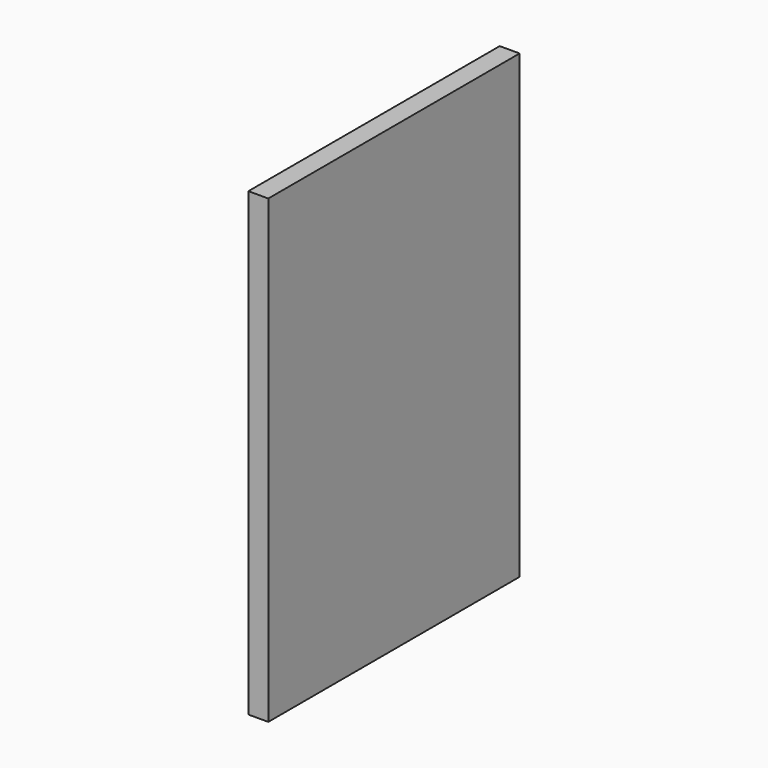
from build123d import *

# Parameters (mm, degrees)
F0_W     = 190.5
F0_H     = 279.4
F2_DEPTH = 12.065


# Not quite as in the source:
# - a variable given as a bare number and used for a length is read in inches; the dataset says mm whatever the document's units were


with BuildPart() as f2:
    # F0 (on Right) → F2 (new body)
    with BuildSketch(Plane.YZ):
        with Locations((95.25, -139.7)):
            Rectangle(F0_W, F0_H)
    extrude(amount=F2_DEPTH)


solid = f2.part
